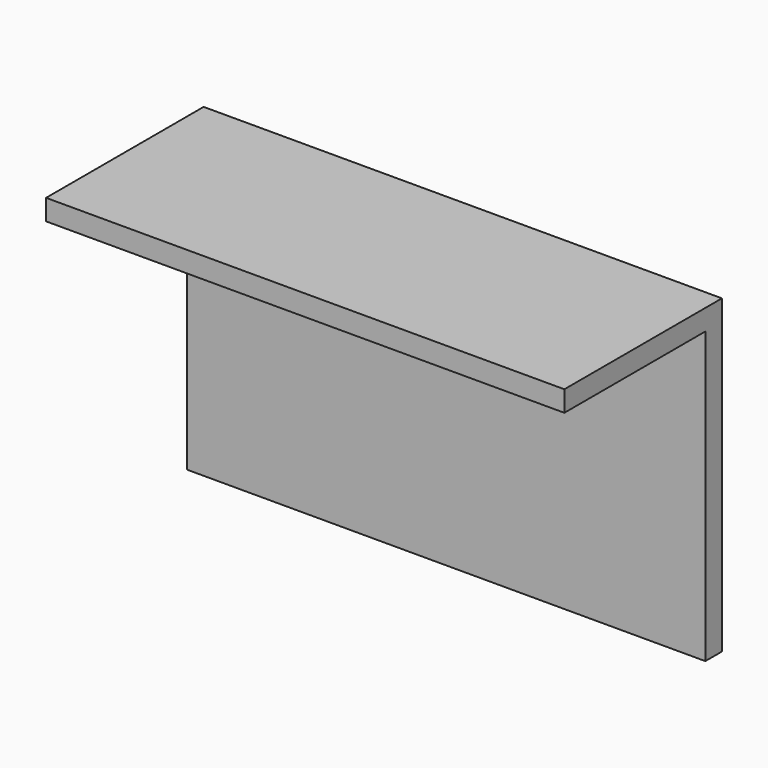
from build123d import *

# Parameters (mm, degrees)
F0_W     = 500
F0_H     = 190
F1_DEPTH = 20
F2_W     = 500
F2_H     = 300
F3_DEPTH = 20


# Not quite as in the source:
# - the program builds the solid bodies; features that only make, move or delete a surface that nothing else refers to are left out


with BuildPart() as f1:
    # F0 (on Top) → F1 (new body)
    with BuildSketch(Plane.XY):
        with Locations((0, -95)):
            Rectangle(F0_W, F0_H)
    extrude(amount=-F1_DEPTH)

    # F2 (on Front) → F3 (join)
    with BuildSketch(Plane.XZ):
        with Locations((0, -150)):
            Rectangle(F2_W, F2_H)
    extrude(amount=F3_DEPTH)


solid = f1.part
